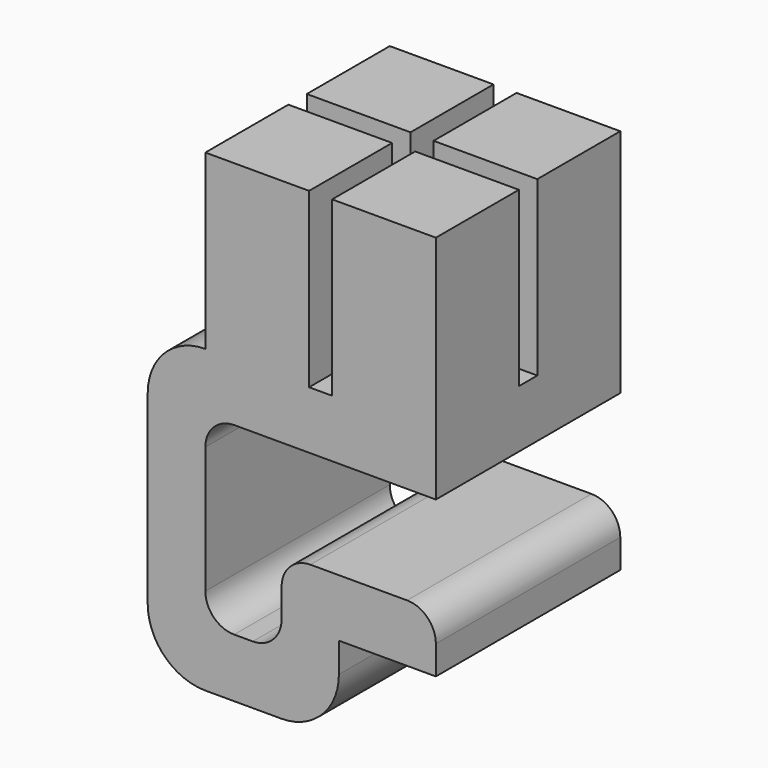
from build123d import *

# Parameters (mm, degrees)
F1_DEPTH = 20
F2_W     = 10
F2_H     = 40
F3_DEPTH = 30
F4_W     = 2
F4_H     = 18
F4_H_2   = 2
F4_W_2   = 18
F5_DEPTH = 30


# Not quite as in the source:
# - a feature names something its author has since deleted; it is built from what else it names


with BuildPart() as f1:
    # F0 (on Front) → F1 (new body, symmetric)
    with BuildSketch(Plane.XZ):
        with BuildLine():
            Line((-10, -5), (20, -5))
            Line((20, -5), (20, 5))
            Line((20, 5), (-20, 5))
            ThreePointArc((-20, 5), (-27.0710678119, 2.0710678119), (-30, -5))
            Line((-30, -5), (-30, -37.0084848255))
            Line((-30, -37.0084848255), (-29.9999700785, -37.1900333921))
            ThreePointArc((-29.9999700785, -37.1900333921), (-27.134358967, -44.1955599538), (-20.1815186475, -47.1867371371))
            Line((-20.1815186475, -47.1867371371), (-20, -47.1900331229))
            Line((-20, -47.1900331229), (-10, -47.1900331229))
            Line((-10, -47.1900331229), (-6.8265195005, -47.1900331229))
            ThreePointArc((-6.8265195005, -47.1900331229), (0.2445483114, -44.2611009348), (3.1734804995, -37.1900331229))
            Line((3.1734804995, -37.1900331229), (3.1734804995, -32.0262350142))
            Line((3.1734804995, -32.0262350142), (20, -32.0262350142))
            Line((20, -32.0262350142), (20, -27.0262350142))
            ThreePointArc((20, -27.0262350142), (18.5355339059, -23.4907011083), (15, -22.0262350142))
            Line((15, -22.0262350142), (3.1734804995, -22.0262350142))
            Line((3.1734804995, -22.0262350142), (-1.7689520504, -22.0262350142))
            ThreePointArc((-1.7689520504, -22.0262350142), (-5.3044859563, -23.4907011083), (-6.7689520504, -27.0262350142))
            Line((-6.7689520504, -27.0262350142), (-6.7689520504, -32.0262350142))
            ThreePointArc((-6.7689520504, -32.0262350142), (-8.2395588674, -35.5501802143), (-11.7686128262, -37.0084848255))
            Line((-11.7686128262, -37.0084848255), (-15, -37.0084848255))
            ThreePointArc((-15, -37.0084848255), (-18.5355339059, -35.5440187314), (-20, -32.0084848255))
            Line((-20, -32.0084848255), (-20, -15))
            Line((-20, -15), (-20, -10))
            ThreePointArc((-20, -10), (-18.5355339059, -6.4644660941), (-15, -5))
            Line((-15, -5), (-10, -5))
        make_face()
    extrude(amount=F1_DEPTH, both=True)

    # F2 (on face) → F3 (join)
    with BuildSketch(Plane.XY.offset(5)):
        with Locations((5, 0)):
            Rectangle(F2_W, F2_H)
        with Locations((-5, 0)):
            Rectangle(F2_W, F2_H)
        with Locations((-15, 0)):
            Rectangle(F2_W, F2_H)
        with Locations((15, 0)):
            Rectangle(F2_W, F2_H)
    extrude(amount=F3_DEPTH)

    # F4 (on face) → F5 (cut)
    with BuildSketch(Plane.XY.offset(35)):
        with Locations((-1, 11)):
            Rectangle(F4_W, F4_H)
        with Locations((-1, 1)):
            Rectangle(F4_W, F4_H_2)
        with Locations((-1, -1)):
            Rectangle(F4_W, F4_H_2)
        with Locations((-1, -11)):
            Rectangle(F4_W, F4_H)
        with Locations((1, 11)):
            Rectangle(F4_W, F4_H)
        with Locations((1, 1)):
            Rectangle(F4_W, F4_H_2)
        with Locations((1, -1)):
            Rectangle(F4_W, F4_H_2)
        with Locations((1, -11)):
            Rectangle(F4_W, F4_H)
        with Locations((11, 1)):
            Rectangle(F4_W_2, F4_H_2)
        with Locations((11, -1)):
            Rectangle(F4_W_2, F4_H_2)
        with Locations((-11, -1)):
            Rectangle(F4_W_2, F4_H_2)
        with Locations((-11, 1)):
            Rectangle(F4_W_2, F4_H_2)
    extrude(amount=-F5_DEPTH, mode=Mode.SUBTRACT)


solid = f1.part
